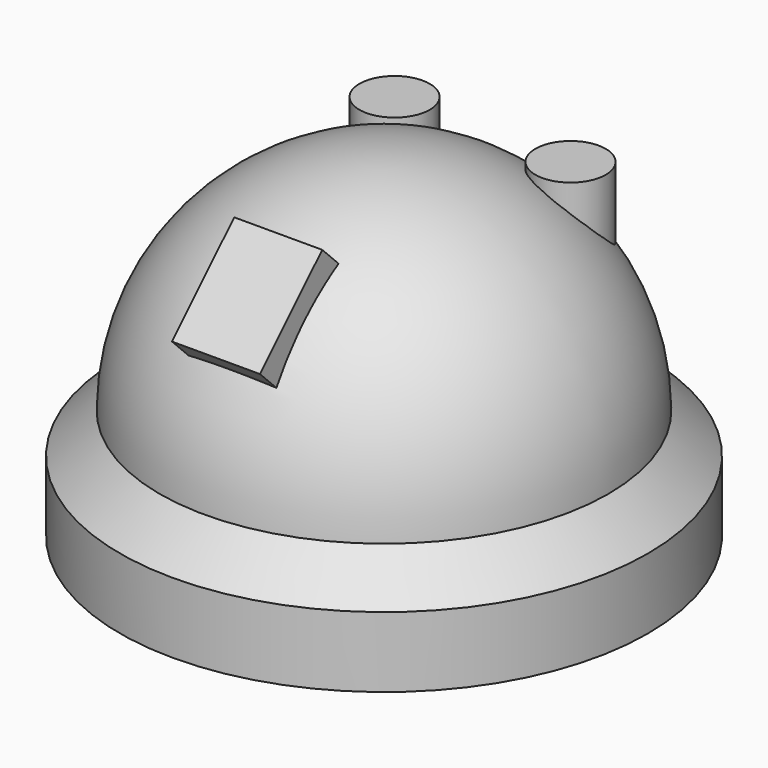
from build123d import *

# Parameters (mm, degrees)
F0_R      = 60
F1_DEPTH  = 25
F2_SIZE   = 9
F6_R      = 8
F7_DEPTH  = 53.9
F12_W     = 20
F12_H     = 25
F13_DEPTH = 35


with BuildPart() as f1:
    # F0 (on Top) → F1 (new body)
    with BuildSketch(Plane.XY):
        Circle(F0_R)
    extrude(amount=F1_DEPTH)

    # F2
    f2_edges = [f1.edges().sort_by_distance(p)[0] for p in [
        (-60, 0, 25),
    ]]
    chamfer(f2_edges, length=F2_SIZE)

    # F3 (on Front) → F4 (revolve)
    with BuildSketch(Plane.XZ):
        with BuildLine():
            Line((0, 25), (51, 25))
            ThreePointArc((51, 25), (36.0624458405, 61.0624458405), (0, 76))
            Line((0, 76), (0, 25))
        make_face()
    revolve(axis=Axis((0, 0, 50.5), (0, 0, 1)))

    # F12 (on face) → F13 (join)
    with BuildSketch(Plane(origin=(0, -51.3908729653, 51.3908729653), x_dir=(1, 0, 0), z_dir=(0, 0.7071067812, -0.7071067812))):
        with Locations((0, -17.6776695297)):
            Rectangle(F12_W, F12_H)
    extrude(amount=F13_DEPTH)


with BuildPart() as f7:
    # F6 (on offset) → F7 (new body)
    with BuildSketch(Plane.XY.offset(70)):
        with Locations((-20, 28)):
            Circle(F6_R)
    extrude(amount=-F7_DEPTH)


with BuildPart() as f7b:
    # F6 (on offset) → F7, piece 2 (new body)
    with BuildSketch(Plane.XY.offset(70)):
        with Locations((20, 28)):
            Circle(F6_R)
    extrude(amount=-F7_DEPTH)


solid = Compound([f1.part, f7.part, f7b.part])
